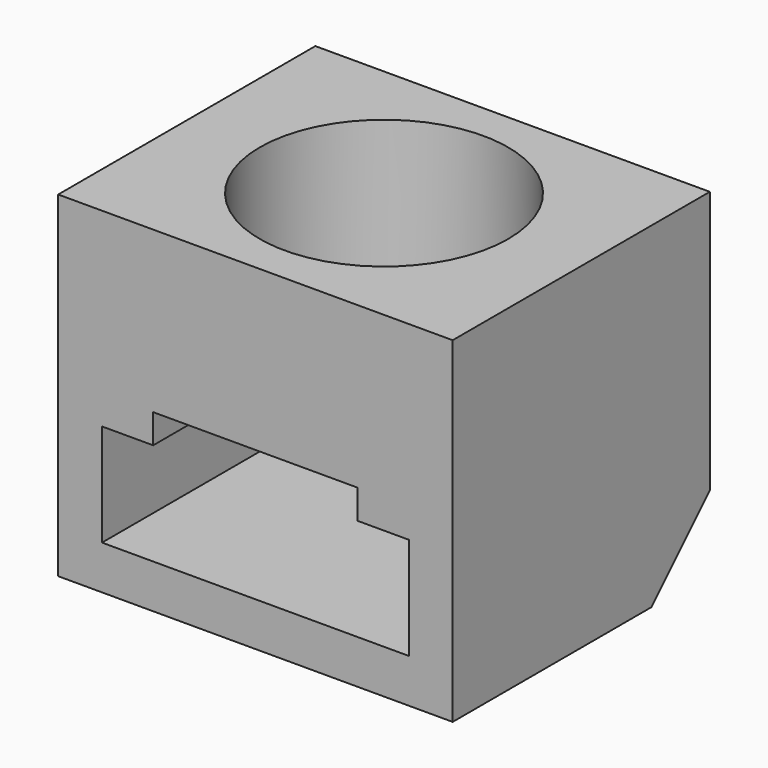
from build123d import *

# Parameters (mm, degrees)
F0_W         = 27
F0_H         = 22
F1_DEPTH     = 20
F2_W         = 21
F2_H         = 21
F3_DEPTH     = 6
F5_DEPTH     = 2
F7_DEPTH     = 20
F8_DEPTH     = 6
F9_W         = 27
F9_H         = 22
F10_DEPTH    = 3
F11_T1_DEPTH = 52.7168298797
F12_R        = 8.5
F13_DEPTH    = 20
F14_DEPTH    = 1


# Not quite as in the source:
# - a fillet or chamfer that OpenCascade refuses, or shapes differently, is made with other operations: its cross-section is extruded or revolved along the edge and cut away or added


with BuildPart() as f1:
    # F0 (on Top) → F1 (new body)
    with BuildSketch(Plane.XY):
        Rectangle(F0_W, F0_H)
    extrude(amount=F1_DEPTH)

    # F2 (on face) → F3 (cut)
    with BuildSketch(Plane(origin=(0, 0, 0), x_dir=(1, 0, 0), z_dir=(0, 0, -1))):
        with Locations((0, 0.5)):
            Rectangle(F2_W, F2_H)
    extrude(amount=-F3_DEPTH, mode=Mode.SUBTRACT)

    # F4 (on face) → F5 (cut)
    with BuildSketch(Plane(origin=(0, 0, 6), x_dir=(1, 0, 0), z_dir=(0, 0, -1))):
        Polygon((0, 11), (-7, 11), (-7, -11), (7, -11), (7, 11), align=None)
    extrude(amount=-F5_DEPTH, mode=Mode.SUBTRACT)

    # F6 (on face) → F7 (cut)
    with BuildSketch(Plane.XY.offset(20)):
        Polygon((0, -3), (3, -3), (3, 3), (-3, 3), (-3, -3), align=None)
    extrude(amount=-F7_DEPTH, mode=Mode.SUBTRACT)

    # F8 (cut): a face of the model
    f8_faces = [f1.faces().sort_by_distance(p)[0] for p in [
        (0, 10.5, 6),
    ]]
    extrude(f8_faces, amount=-F8_DEPTH, mode=Mode.SUBTRACT)

    # F9 (on face) → F10 (join)
    with BuildSketch(Plane(origin=(0, 0, 0), x_dir=(1, 0, 0), z_dir=(0, 0, -1))):
        Rectangle(F9_W, F9_H)
    extrude(amount=F10_DEPTH)

    # F11: chamfer of 5 on 1 edges, made by hand

    # F11_s2 → F11_t1 (cut)
    with BuildSketch(Plane.YZ.offset(-26.3584149398)):
        Polygon((11, 2), (6, -3), (11, -3), align=None)
    extrude(amount=F11_T1_DEPTH, mode=Mode.SUBTRACT)

    # F12 (on face) → F13 (cut)
    with BuildSketch(Plane.XY.offset(20)):
        Circle(F12_R)
    extrude(amount=-F13_DEPTH, mode=Mode.SUBTRACT)

    # F14 (cut): faces of the model
    f14_faces = [f1.faces().sort_by_distance(p)[0] for p in [
        (-8.9267642555, -0.5771749807, 6),
        (8.9267642555, -0.5771749807, 6),
        (0, -9.0505273171, 8),
        (0, 9.0505273171, 8),
    ]]
    extrude(f14_faces, amount=-F14_DEPTH, mode=Mode.SUBTRACT)


solid = f1.part
